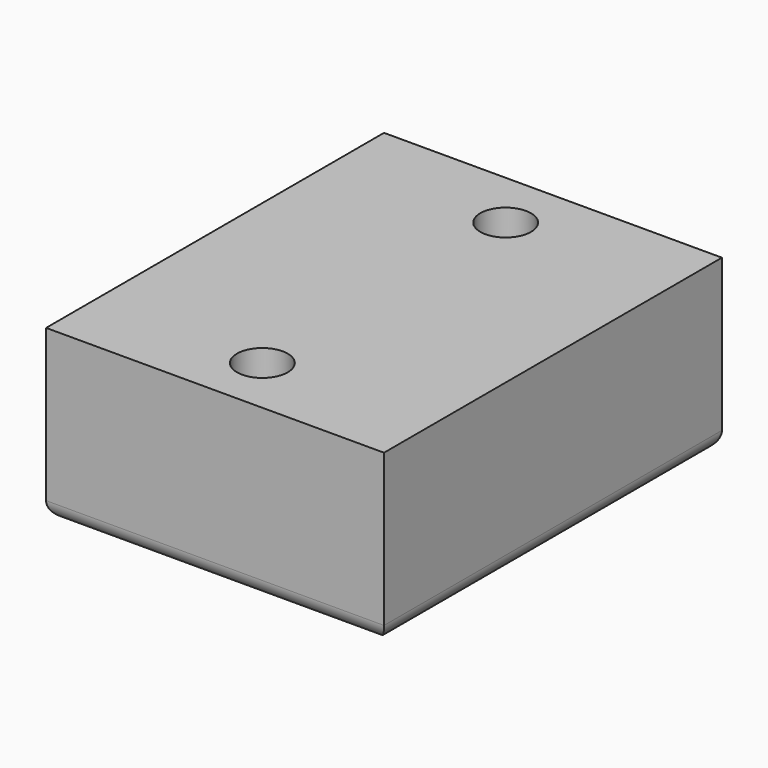
from build123d import *

# Parameters (mm, degrees)
F0_W     = 20
F0_H     = 25
F1_DEPTH = 10
F3_D     = 3
F3_DEPTH = 10
F3_TIP   = 0.9012909285
F4_R     = 0.99999


# Not quite as in the source:
# - a fillet or chamfer is up to 0.001 mm smaller than in the source, because OpenCascade refuses the exact size


with BuildPart() as f1:
    # F0 (on Top) → F1 (new body)
    with BuildSketch(Plane.XY):
        with Locations((-11.3712290768, -0.8075441738)):
            Rectangle(F0_W, F0_H)
    extrude(amount=F1_DEPTH)

    # F3
    with Locations(Plane.XY.offset(10)):
        with Locations((-11.3712290768, 8.1924558262), (-11.3712290768, -9.8075441738)):
            Hole(F3_D / 2, depth=F3_DEPTH)
            with Locations((0, 0, -(F3_DEPTH + F3_TIP / 2))):  # 118° drill point
                Cone(0, F3_D / 2, F3_TIP, mode=Mode.SUBTRACT)

    # F4 (radius 1 in the source; OpenCascade refuses exactly that, so slightly less here)
    f4_edges = [f1.edges().sort_by_distance(p)[0] for p in [
        (-11.371229, -13.307544, 0),
        (-21.371229, -0.807544, 0),
        (-1.371229, -0.807544, 0),
        (-11.371229, 11.692456, 0),
        (-12.871229, -9.807544, 0),
        (-12.871229, 8.192456, 0),
    ]]
    fillet(f4_edges, radius=F4_R)


solid = f1.part
